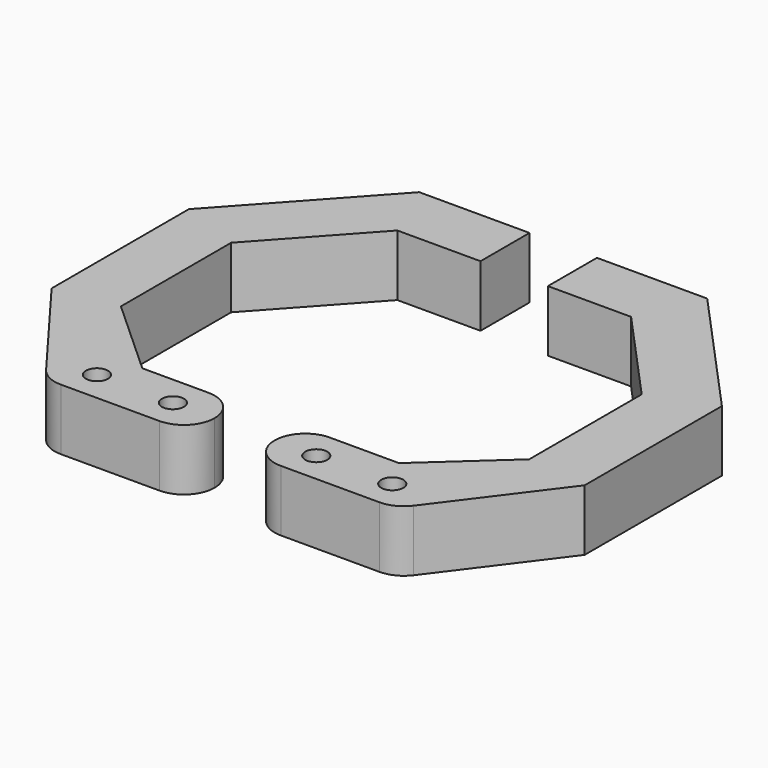
from build123d import *

# Parameters (mm, degrees)
F0_R     = 1.8
F1_DEPTH = 10
F2_R     = 4.99999
F2_2_R   = 4.99999
F3_R     = 5
F3_2_R   = 5


# Not quite as in the source:
# - a fillet or chamfer is up to 0.001 mm smaller than in the source, because OpenCascade refuses the exact size


with BuildPart() as f1:
    # F0 (on Top) → F1 (new body)
    with BuildSketch(Plane.XY):
        Polygon((4.8827224633, -32.8996852207), (28.4827224633, -32.8996852207), (43.4827224633, -12.8996852207), (43.4827224633, 15.1003147793), (23.4827224633, 37.1003147793), (5.4827224633, 37.1003147793), (5.4827224633, 27.1003147793), (19.0590236021, 27.1003147793), (33.4827224633, 11.234246032), (33.4827224633, -11.7159301209), (21.1805918535, -22.8996852207), (4.8827224633, -22.8996852207), align=None)
        with Locations((11.6827224633, -27.8996852207)):
            Circle(F0_R, mode=Mode.SUBTRACT)
        with Locations((24.0827224633, -27.8996852207)):
            Circle(F0_R, mode=Mode.SUBTRACT)
    extrude(amount=F1_DEPTH)

    # F2#2 (radius 5 in the source; OpenCascade refuses exactly that, so slightly less here)
    f2_2_edges = [f1.edges().sort_by_distance(p)[0] for p in [
        (4.882722, -22.899685, 5),
        (4.882722, -32.899685, 5),
    ]]
    fillet(f2_2_edges, radius=F2_2_R)

    # F3#2
    f3_2_edges = [f1.edges().sort_by_distance(p)[0] for p in [
        (28.482722, -32.899685, 5),
    ]]
    fillet(f3_2_edges, radius=F3_2_R)


with BuildPart() as f1b:
    # F0 (on Top) → F1, piece 2 (new body)
    with BuildSketch(Plane.XY):
        Polygon((-43.5172775367, 15.1003147793), (-43.5172775367, -12.8996852207), (-28.5172775367, -32.8996852207), (-4.9172775367, -32.8996852207), (-4.9172775367, -22.8996852207), (-20.7140983621, -22.8996852207), (-33.5172775367, -11.2604314256), (-33.5172775367, 11.234246032), (-19.0935786755, 27.1003147793), (-5.5172775367, 27.1003147793), (-5.5172775367, 37.1003147793), (-23.5172775367, 37.1003147793), align=None)
        with Locations((-24.1172775367, -27.8996852207)):
            Circle(F0_R, mode=Mode.SUBTRACT)
        with Locations((-11.7172775367, -27.8996852207)):
            Circle(F0_R, mode=Mode.SUBTRACT)
    extrude(amount=F1_DEPTH)

    # F2 (radius 5 in the source; OpenCascade refuses exactly that, so slightly less here)
    f2_edges = [f1b.edges().sort_by_distance(p)[0] for p in [
        (-4.917278, -32.899685, 5),
        (-4.917278, -22.899685, 5),
    ]]
    fillet(f2_edges, radius=F2_R)

    # F3
    f3_edges = [f1b.edges().sort_by_distance(p)[0] for p in [
        (-28.517278, -32.899685, 5),
    ]]
    fillet(f3_edges, radius=F3_R)


solid = Compound([f1.part, f1b.part])
